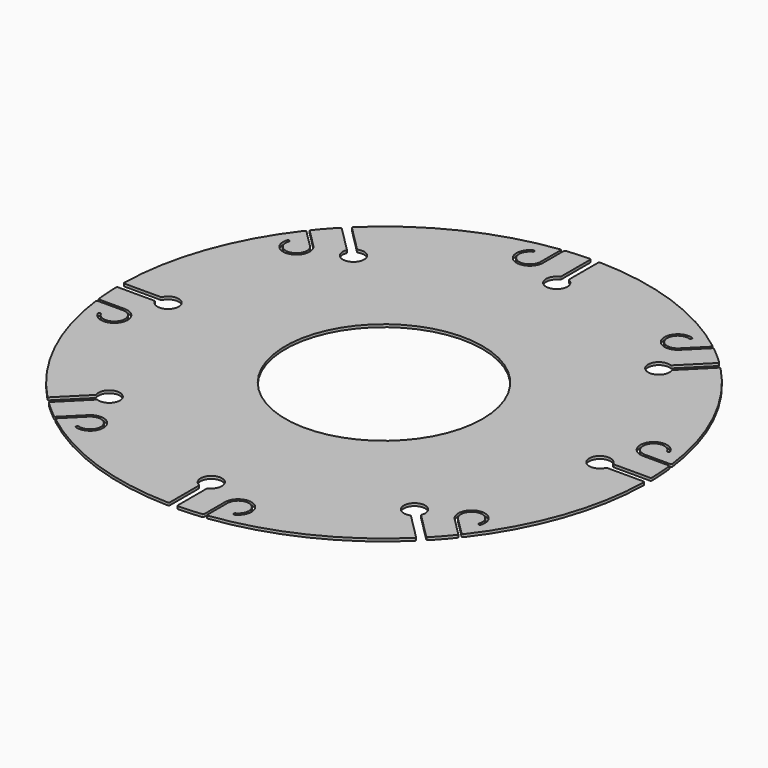
from build123d import *

# Parameters (mm, degrees)
F0_R            = 185
F2_DEPTH        = 5
F3_DEPTH        = 5
F3_COPIES_COUNT = 8
F4_R            = 2


# Not quite as in the source:
# - a pattern or mirror of a feature is missing from the dataset's text; its kind, count and spacing are read off the source's solid
# - a feature names something its author has since deleted; it is built from what else it names


with BuildPart() as f2:
    # F0 (on Top) → F2 (new body)
    with BuildSketch(Plane.XY):
        with BuildLine():
            ThreePointArc((-491.3501806248, -60), (30.055453671, -494.0867026187), (495, 0))
            ThreePointArc((495, 0), (3.750107621, 494.9857944354), (-494.9431785569, 7.5))
            Line((-494.9431785569, 7.5), (-424.843134833, 7.5))
            ThreePointArc((-424.843134833, 7.5), (-423.7771312512, 7.8077717755), (-423.0392134845, 8.6363636364))
            ThreePointArc((-423.0392134845, 8.6363636364), (-385, 0), (-423.0392134845, -8.6363636364))
            ThreePointArc((-423.0392134845, -8.6363636364), (-423.7771312512, -7.8077717755), (-424.843134833, -7.5))
            Line((-424.843134833, -7.5), (-494.9431785569, -7.5))
            ThreePointArc((-494.9431785569, -7.5), (-494.0102986253, -31.2861766946), (-491.93495505, -55))
            Line((-491.93495505, -55), (-441.93495505, -55))
            ThreePointArc((-441.93495505, -55), (-420.5886816099, -93.0129401067), (-464.1571772722, -91.4530711823))
            ThreePointArc((-464.1571772722, -91.4530711823), (-463.0802621682, -88.0855418418), (-459.7127328277, -89.1624569458))
            ThreePointArc((-459.7127328277, -89.1624569458), (-424.8579362979, -90.4103520854), (-441.93495505, -60))
            Line((-441.93495505, -60), (-491.3501806248, -60))
        make_face()
        Circle(F0_R, mode=Mode.SUBTRACT)
        with BuildLine():
            Line((-424.843134833, 7.5), (-494.9431785569, 7.5))
            ThreePointArc((-494.9431785569, 7.5), (-495, 0), (-494.9431785569, -7.5))
            Line((-494.9431785569, -7.5), (-424.843134833, -7.5))
            ThreePointArc((-424.843134833, -7.5), (-423.7771312512, -7.8077717755), (-423.0392134845, -8.6363636364))
            ThreePointArc((-423.0392134845, -8.6363636364), (-385, 0), (-423.0392134845, 8.6363636364))
            ThreePointArc((-423.0392134845, 8.6363636364), (-423.7771312512, 7.8077717755), (-424.843134833, 7.5))
        make_face()
        with BuildLine():
            ThreePointArc((-491.93495505, -55), (-491.64892404, -57.500743389), (-491.3501806248, -60))
            Line((-491.3501806248, -60), (-441.93495505, -60))
            ThreePointArc((-441.93495505, -60), (-424.8579362979, -90.4103520854), (-459.7127328277, -89.1624569458))
            ThreePointArc((-459.7127328277, -89.1624569458), (-463.0802621682, -88.0855418418), (-464.1571772722, -91.4530711823))
            ThreePointArc((-464.1571772722, -91.4530711823), (-420.5886816099, -93.0129401067), (-441.93495505, -55))
            Line((-441.93495505, -55), (-491.93495505, -55))
        make_face()
    extrude(amount=F2_DEPTH)

    # F0 (on Top) → F3 (cut, through all)
    with BuildSketch(Plane.XY):
        with BuildLine():
            Line((-424.843134833, 7.5), (-494.9431785569, 7.5))
            ThreePointArc((-494.9431785569, 7.5), (-495, 0), (-494.9431785569, -7.5))
            Line((-494.9431785569, -7.5), (-424.843134833, -7.5))
            ThreePointArc((-424.843134833, -7.5), (-423.7771312512, -7.8077717755), (-423.0392134845, -8.6363636364))
            ThreePointArc((-423.0392134845, -8.6363636364), (-385, 0), (-423.0392134845, 8.6363636364))
            ThreePointArc((-423.0392134845, 8.6363636364), (-423.7771312512, 7.8077717755), (-424.843134833, 7.5))
        make_face()
        with BuildLine():
            ThreePointArc((-491.93495505, -55), (-491.64892404, -57.500743389), (-491.3501806248, -60))
            Line((-491.3501806248, -60), (-441.93495505, -60))
            ThreePointArc((-441.93495505, -60), (-424.8579362979, -90.4103520854), (-459.7127328277, -89.1624569458))
            ThreePointArc((-459.7127328277, -89.1624569458), (-463.0802621682, -88.0855418418), (-464.1571772722, -91.4530711823))
            ThreePointArc((-464.1571772722, -91.4530711823), (-420.5886816099, -93.0129401067), (-441.93495505, -55))
            Line((-441.93495505, -55), (-491.93495505, -55))
        make_face()
    f3 = extrude(amount=F3_DEPTH, mode=Mode.SUBTRACT)

    # F3_copies: F3 ×8 about axis
    f3_copies_axis = Axis((0, 0, 0), (0, 0, 1))
    for i in range(1, F3_COPIES_COUNT):
        add(f3.rotate(f3_copies_axis, i * 360 / F3_COPIES_COUNT), mode=Mode.SUBTRACT)

    # F4
    f4_edges = [f2.edges().sort_by_distance(p)[0] for p in [
        (-494.943179, -7.5, 2.5),
        (-494.943179, 7.5, 2.5),
        (-491.934955, -55, 2.5),
        (-491.350181, -60, 2.5),
        (-355.280979, -344.674377, 2.5),
        (-389.863452, 305.010638, 2.5),
        (-386.741416, 308.95967, 2.5),
        (-355.280979, 344.674377, 2.5),
        (-344.674377, 355.280979, 2.5),
        (-60, 491.350181, 2.5),
        (-55, 491.934955, 2.5),
        (-7.5, 494.943179, 2.5),
        (7.5, 494.943179, 2.5),
        (305.010638, 389.863452, 2.5),
        (308.95967, 386.741416, 2.5),
        (344.674377, 355.280979, 2.5),
        (355.280979, 344.674377, 2.5),
        (491.350181, 60, 2.5),
        (491.934955, 55, 2.5),
        (494.943179, 7.5, 2.5),
        (494.943179, -7.5, 2.5),
        (389.863452, -305.010638, 2.5),
        (386.741416, -308.95967, 2.5),
        (355.280979, -344.674377, 2.5),
        (344.674377, -355.280979, 2.5),
        (60, -491.350181, 2.5),
        (55, -491.934955, 2.5),
        (7.5, -494.943179, 2.5),
        (-7.5, -494.943179, 2.5),
        (-305.010638, -389.863452, 2.5),
        (-308.95967, -386.741416, 2.5),
        (-344.674377, -355.280979, 2.5),
    ]]
    fillet(f4_edges, radius=F4_R)


solid = f2.part
